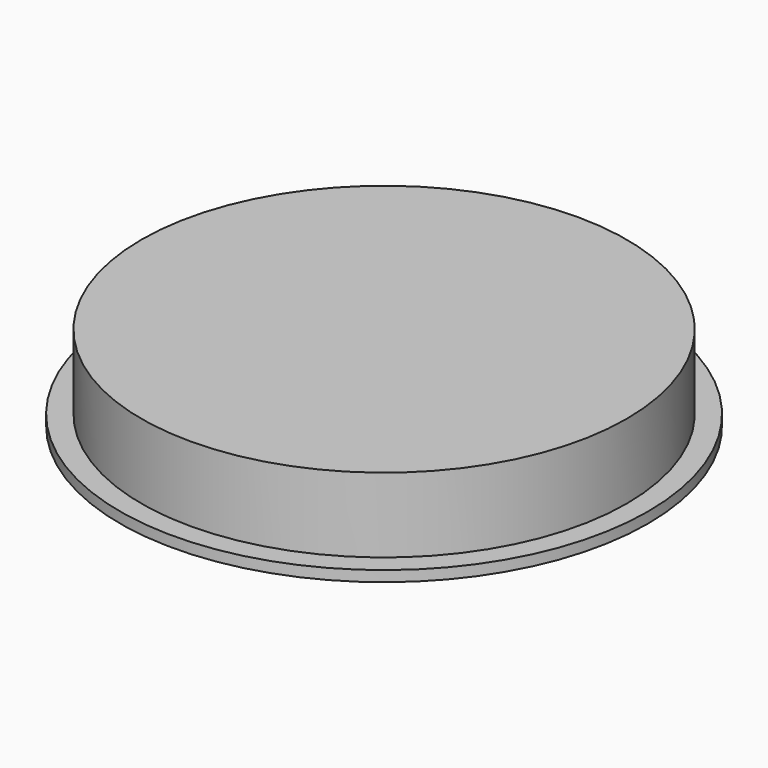
from build123d import *

# Parameters (mm, degrees)
F0_R     = 24.75
F0_R_2   = 22.75
F1_DEPTH = 1
F0_R_3   = 21.75
F0_R_4   = 20.75
F2_DEPTH = 8
F3_T     = 1


# Not quite as in the source:
# - a shell that OpenCascade refuses in one call is made with other operations: the cavity is built on its own and cut out


with BuildPart() as f1:
    # F0 (on Top) → F1 (new body)
    with BuildSketch(Plane.XY):
        with Locations((-30.0056487322, 13.6389313266)):
            Circle(F0_R)
        with Locations((-30.0056487322, 13.6389313266)):
            Circle(F0_R_2, mode=Mode.SUBTRACT)
    extrude(amount=F1_DEPTH)

    # F0 (on Top) → F2 (join)
    with BuildSketch(Plane.XY):
        with Locations((-30.0056487322, 13.6389313266)):
            Circle(F0_R_2)
        with Locations((-30.0056487322, 13.6389313266)):
            Circle(F0_R_3, mode=Mode.SUBTRACT)
        with Locations((-30.0056487322, 13.6389313266)):
            Circle(F0_R_3)
        with Locations((-30.0056487322, 13.6389313266)):
            Circle(F0_R_4, mode=Mode.SUBTRACT)
        with Locations((-30.0056487322, 13.6389313266)):
            Circle(F0_R_4)
    extrude(amount=F2_DEPTH)

    # F3: shell of thickness 1, made by hand


with BuildPart() as f3_core1:
    # F3_t2: copy of F1
    add(f1.part)

    # the walls: a layer under each face that stays
    f3_faces = [f3_core1.faces().sort_by_distance(p)[0] for p in [
        (-54.7556487322, 13.6389313266, 0.5),
        (-46.5056487322, -2.8610686734, 1),
        (-52.7556487322, 13.6389313266, 4.5),
        (-30.0056487322, 13.6389313266, 8),
    ]]
    thicken(f3_faces, amount=-F3_T, mode=Mode.SUBTRACT)

    # F3_s3 → F3_t4 (revolve, cut)
    with BuildSketch(Plane.XZ.offset(-13.6389313266)):
        Polygon((-7.2456487322, 1.01), (-7.2556487322, 0), (-8.2556487322, 0), (-8.2556487322, 1), align=None)
    revolve(axis=Axis((-30.0056487322, 13.6389313266, 1), (0, 0, 1)), mode=Mode.SUBTRACT)


with BuildPart() as f1_1:
    add(f1.part)

    # what is left inside the walls is the cavity
    f3_cavity = [f3_core1.part.solids().sort_by_distance(p)[0] for p in [
        (-30.005649, 6.388931, 6.99),
    ]]
    add(f3_cavity, mode=Mode.SUBTRACT)


solid = f1_1.part
